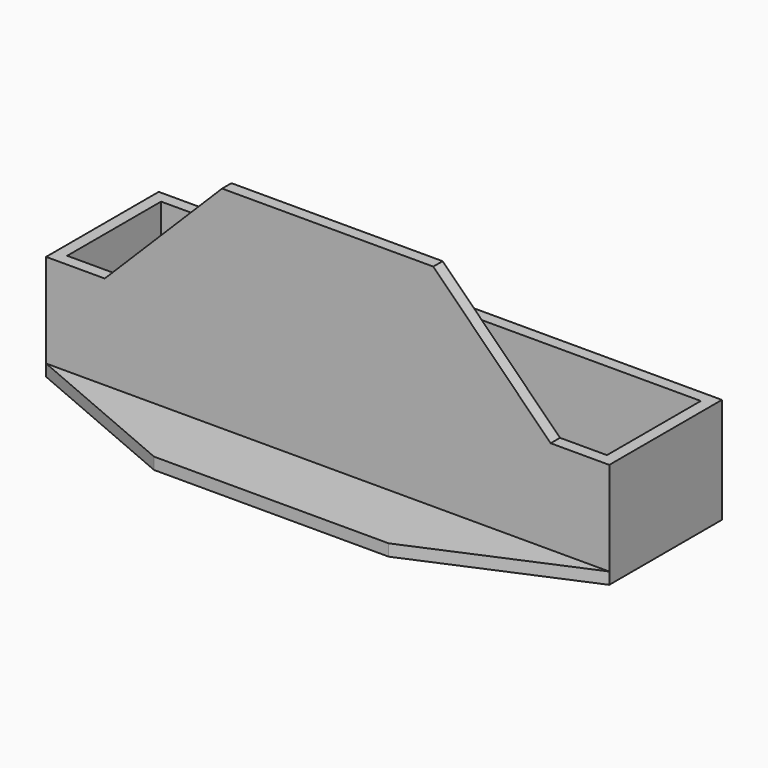
from build123d import *

# Parameters (mm, degrees)
F0_W     = 96
F0_H     = 24
F1_DEPTH = 2
F2_W     = 36
F2_H     = 2
F3_DEPTH = 36
F2_W_2   = 92
F2_W_3   = 2
F2_H_2   = 20
F2_W_4   = 28
F4_DEPTH = 16
F5_SIZE  = 19.99999
F6_DEPTH = 2


# Not quite as in the source:
# - a fillet or chamfer is up to 0.001 mm smaller than in the source, because OpenCascade refuses the exact size


with BuildPart() as f1:
    # F0 (on Top) → F1 (new body)
    with BuildSketch(Plane.XY):
        with Locations((48, 12)):
            Rectangle(F0_W, F0_H)
    extrude(amount=F1_DEPTH)

    # F2 (on face) → F3 (join)
    with BuildSketch(Plane.XY.offset(2)):
        with Locations((48, 1)):
            Rectangle(F2_W, F2_H)
    extrude(amount=F3_DEPTH)

    # F2 (on face) → F4 (join)
    with BuildSketch(Plane.XY.offset(2)):
        with Locations((48, 23)):
            Rectangle(F2_W_2, F2_H)
        with Locations((95, 23)):
            Rectangle(F2_W_3, F2_H)
        with Locations((48, 1)):
            Rectangle(F2_W, F2_H)
        with Locations((95, 12)):
            Rectangle(F2_W_3, F2_H_2)
        with Locations((95, 1)):
            Rectangle(F2_W_3, F2_H)
        Polygon((2, 22), (2, 24), (0, 24), (0, 2), (2, 2), align=None)
        with Locations((1, 1)):
            Rectangle(F2_W_3, F2_H)
        with Locations((16, 1)):
            Rectangle(F2_W_4, F2_H)
        with Locations((80, 1)):
            Rectangle(F2_W_4, F2_H)
    extrude(amount=F4_DEPTH)

    # F5 (size 20 in the source; OpenCascade refuses exactly that, so slightly less here)
    f5_edges = [f1.edges().sort_by_distance(p)[0] for p in [
        (30, 1, 18),
        (66, 1, 18),
    ]]
    chamfer(f5_edges, length=F5_SIZE)

    # F0 (on Top) → F6 (join, through all)
    with BuildSketch(Plane.XY):
        Polygon((96, 0), (0, 0), (28, -12), (68, -12), align=None)
    extrude(amount=F6_DEPTH)


solid = f1.part
